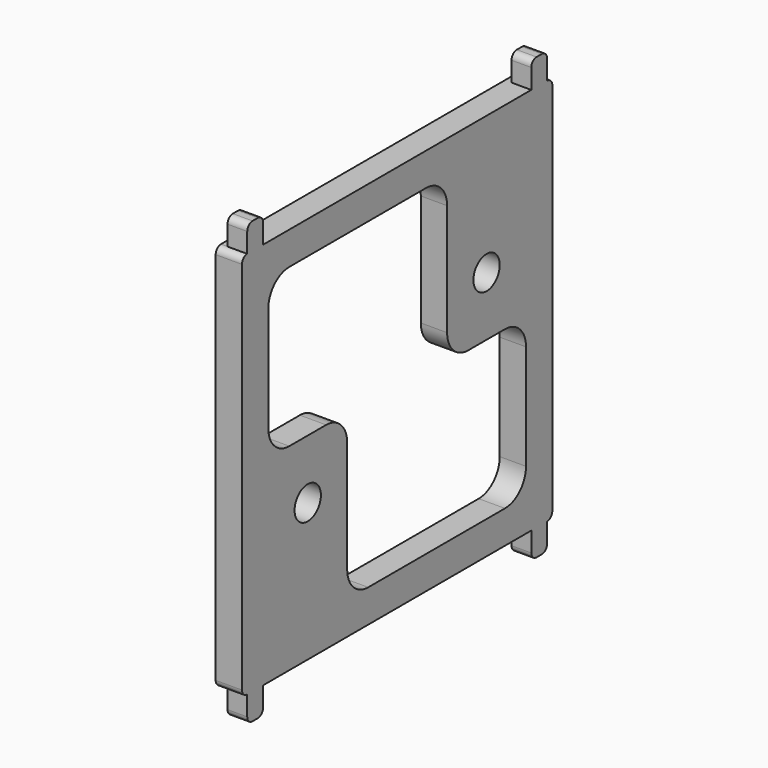
from build123d import *

# Parameters (mm, degrees)
F0_W     = 3
F0_H     = 4
F0_W_2   = 15
F0_H_2   = 25
F0_R     = 2.5
F1_DEPTH = 4
F2_W     = 3
F2_H     = 4
F3_DEPTH = 1
F4_R     = 4
F5_R     = 0.99999


# Not quite as in the source:
# - a fillet or chamfer is up to 0.001 mm smaller than in the source, because OpenCascade refuses the exact size


with BuildPart() as f1:
    # F0 (on Right) → F1 (new body)
    with BuildSketch(Plane.YZ):
        Polygon((-28.5, 29.5), (-29.5, 29.5), (-29.5, -29.5), (-28.5, -29.5), (-25.5, -29.5), (25.5, -29.5), (28.5, -29.5), (29.5, -29.5), (29.5, 29.5), (28.5, 29.5), (25.5, 29.5), (-25.5, 29.5), align=None)
        Polygon((-24.5, 0.5), (-24.5, 24.5), (9.5, 24.5), (24.5, 24.5), (24.5, -0.5), (24.5, -24.5), (-9.5, -24.5), (-24.5, -24.5), align=None, mode=Mode.SUBTRACT)
        with Locations((-27, 31.5)):
            Rectangle(F0_W, F0_H)
        with Locations((27, 31.5)):
            Rectangle(F0_W, F0_H)
        with Locations((-27, -31.5)):
            Rectangle(F0_W, F0_H)
        with Locations((27, -31.5)):
            Rectangle(F0_W, F0_H)
        with Locations((-17, -12)):
            Rectangle(F0_W_2, F0_H_2)
        with Locations((-17, -8.5)):
            Circle(F0_R, mode=Mode.SUBTRACT)
        with Locations((17, 12)):
            Rectangle(F0_W_2, F0_H_2)
        with Locations((17, 8.5)):
            Circle(F0_R, mode=Mode.SUBTRACT)
    extrude(amount=F1_DEPTH)

    # F2 (on face) → F3 (cut)
    with BuildSketch(Plane(origin=(0, 0, 0), x_dir=(0, -1, 0), z_dir=(-1, 0, 0))):
        with Locations((-27, 31.5)):
            Rectangle(F2_W, F2_H)
        with Locations((27, 31.5)):
            Rectangle(F2_W, F2_H)
        with Locations((-27, -31.5)):
            Rectangle(F2_W, F2_H)
        with Locations((27, -31.5)):
            Rectangle(F2_W, F2_H)
    extrude(amount=-F3_DEPTH, mode=Mode.SUBTRACT)

    # F4
    f4_edges = [f1.edges().sort_by_distance(p)[0] for p in [
        (2, 9.5, -0.5),
        (2, 9.5, 24.5),
        (2, 24.5, -0.5),
        (2, -9.5, 0.5),
        (2, -24.5, 0.5),
        (2, -9.5, -24.5),
        (2, -24.5, 24.5),
        (2, 24.5, -24.5),
    ]]
    fillet(f4_edges, radius=F4_R)

    # F5 (radius 1 in the source; OpenCascade refuses exactly that, so slightly less here)
    f5_edges = [f1.edges().sort_by_distance(p)[0] for p in [
        (2.5, 28.5, 33.5),
        (2.5, 25.5, 33.5),
        (2.5, -25.5, 33.5),
        (2.5, -28.5, 33.5),
        (2, 29.5, 29.5),
        (2, -29.5, 29.5),
        (2, -29.5, -29.5),
        (2.5, -28.5, -33.5),
        (2.5, -25.5, -33.5),
        (2, 29.5, -29.5),
        (2.5, 28.5, -33.5),
        (2.5, 25.5, -33.5),
    ]]
    fillet(f5_edges, radius=F5_R)


solid = f1.part
